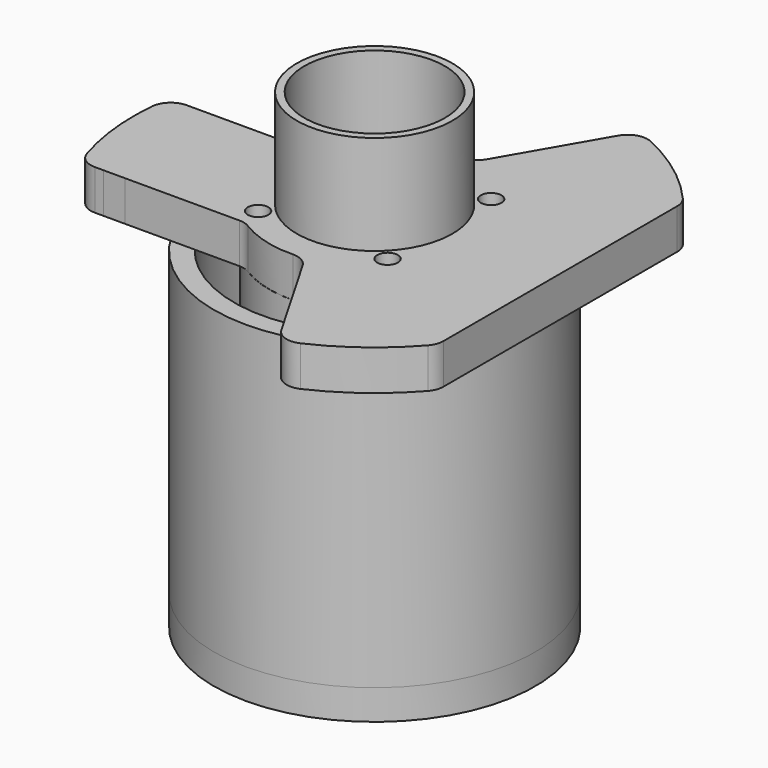
from build123d import *

# Parameters (mm, degrees)
F0_W      = 12.7
F0_H      = 12.86002
F0_R      = 11.1125
F0_H_2    = 0.00127
F1_DEPTH  = 6.35
F12_D     = 2.4384
F12_DEPTH = 4.7625
F12_TIP   = 0.7325692667
F11_R     = 21.63445
F11_R_2   = 14.478
F13_DEPTH = 1.190625
F14_D     = 2.4384
F16_D     = 2.2606
F16_DEPTH = 6.35
F16_TIP   = 0.6791527577
F17_D     = 3.2639


# Not quite as in the source:
# - a feature names something its author has since deleted; it is built from what else it names


with BuildPart() as f1:
    # F0 (on Top) → F1 (new body)
    with BuildSketch(Plane.XY):
        with BuildLine():
            ThreePointArc((29.36875, 23.1007161347), (29.1636905508, 24.2232481499), (28.575, 25.2007812379))
            ThreePointArc((28.575, 25.2007812379), (22.762711603, 30.5527242726), (15.9715205932, 34.5907578688))
            ThreePointArc((15.9715205932, 34.5907578688), (13.6801160021, 34.7344417755), (11.8909298868, 33.2956947131))
            Line((11.8909298868, 33.2956947131), (3.1737490765, 18.197094651))
            ThreePointArc((3.1737490765, 18.197094651), (1.9820606936, 17.0181093591), (0.3560722092, 16.6103239138))
            ThreePointArc((0.3560722092, 16.6103239138), (-8.30707, 14.388267302), (-14.5629985791, 7.9967943781))
            ThreePointArc((-14.5629985791, 7.9967943781), (-15.7291453761, 6.792539767), (-17.3460207811, 6.35))
            Line((-17.3460207811, 6.35), (-34.7803824016, 6.35))
            ThreePointArc((-34.7803824016, 6.35), (-36.9209669649, 5.5198929032), (-37.9422353472, 3.4636363636))
            ThreePointArc((-37.9422353472, 3.4636363636), (-37.8826451562, -4.0638892662), (-36.3442120473, -11.4327709091))
            ThreePointArc((-36.3442120473, -11.4327709091), (-35.1937854617, -13.039878436), (-33.31552771, -13.65504))
            Line((-33.31552771, -13.65504), (-31.9626256824, -13.65377))
            Line((-31.9626256824, -13.65377), (-28.575, -13.65377))
            Line((-28.575, -13.65377), (-28.575, -6.35))
            Line((-28.575, -6.35), (-28.575, -0.79375))
            Line((-28.575, -0.79375), (-15.875, -0.79375))
            Line((-15.875, -0.79375), (-15.875, -13.65377))
            Line((-15.875, -13.65377), (-15.875, -13.65504))
            Line((-15.875, -13.65504), (-10.4096020836, -13.65504))
            ThreePointArc((-10.4096020836, -13.65504), (-9.5414514384, -13.7760361596), (-8.7394695454, -14.1298025465))
            ThreePointArc((-8.7394695454, -14.1298025465), (-4.3713366706, -16.0287573958), (0.3560722092, -16.6103239138))
            ThreePointArc((0.3560722092, -16.6103239138), (1.9820606936, -17.0181093591), (3.1737490765, -18.197094651))
            Line((3.1737490765, -18.197094651), (11.8909298868, -33.2956947131))
            ThreePointArc((11.8909298868, -33.2956947131), (13.6801160021, -34.7344417755), (15.9715205932, -34.5907578688))
            ThreePointArc((15.9715205932, -34.5907578688), (22.762711603, -30.5527242726), (28.575, -25.2007812379))
            ThreePointArc((28.575, -25.2007812379), (29.1636905508, -24.2232481499), (29.36875, -23.1007161347))
            Line((29.36875, -23.1007161347), (29.36875, 23.1007161347))
        make_face()
        with Locations((22.225, -7.22376)):
            Rectangle(F0_W, F0_H, mode=Mode.SUBTRACT)
        Circle(F0_R, mode=Mode.SUBTRACT)
        with Locations((-22.225, -13.654405)):
            Rectangle(F0_W, F0_H_2)
        Polygon((-28.575, -13.65377), (-15.875, -13.65377), (-15.875, -0.79375), (-28.575, -0.79375), (-28.575, -6.35), align=None)
        with Locations((22.225, -7.22376)):
            Rectangle(F0_W, F0_H)
    extrude(amount=F1_DEPTH)

    # F17 (through all)
    with Locations(Plane(origin=(0, 0, 0), x_dir=(1, 0, 0), z_dir=(0, 0, -1))):
        with Locations((-10.237491978, -10.237491978), (10.237491978, -10.237491978), (10.237491978, 10.237491978), (-10.237491978, 10.237491978)):
            Hole(F17_D / 2)


with BuildPart() as f6:
    # F5 (on Right) → F6 (revolve)
    with BuildSketch(Plane.YZ):
        Polygon((12.303125, 22.08276), (11.1125, 22.08276), (11.1125, -26.91638), (13.462, -26.91638), (13.462, -25.725755), (12.303125, -25.725755), align=None)
    revolve(axis=Axis((0, 0, -24.5783533533), (0, 0, -1)))


with BuildPart() as f8:
    # F7 (on Right) → F8 (revolve)
    with BuildSketch(Plane.YZ):
        with BuildLine():
            Line((13.462, -25.725755), (13.462, -26.91638))
            Line((13.462, -26.91638), (13.462, -49.2125))
            Line((13.462, -49.2125), (14.1478, -49.2125))
            ThreePointArc((14.1478, -49.2125), (15.0368, -48.3235), (15.9258, -49.2125))
            Line((15.9258, -49.2125), (16.891, -49.2125))
            Line((16.891, -49.2125), (16.891, -52.3875))
            Line((16.891, -52.3875), (25.4, -52.3875))
            Line((25.4, -52.3875), (25.4, -47.625))
            Line((25.4, -47.625), (22.225, -47.625))
            Line((22.225, -47.625), (22.225, -42.8625))
            Line((22.225, -42.8625), (16.637, -42.8625))
            Line((16.637, -42.8625), (16.637, 0))
            Line((16.637, 0), (12.303125, 0))
            Line((12.303125, 0), (12.303125, -25.725755))
            Line((12.303125, -25.725755), (13.462, -25.725755))
        make_face()
    revolve(axis=Axis((0, 0, -24.60625), (0, 0, -1)))

    # F12
    with Locations(Plane(origin=(0, 0, -52.3875), x_dir=(1, 0, 0), z_dir=(0, 0, -1))):
        with Locations((-18.4785, 0), (9.23925, 16.0028504238), (18.4785, 0), (9.23925, -16.0028504238), (-9.23925, -16.0028504238), (-9.23925, 16.0028504238)):
            Hole(F12_D / 2, depth=F12_DEPTH)
            with Locations((0, 0, -(F12_DEPTH + F12_TIP / 2))):  # 118° drill point
                Cone(0, F12_D / 2, F12_TIP, mode=Mode.SUBTRACT)

    # F16
    with Locations(Plane.XY):
        with Locations((-10.237491978, 10.237491978), (10.237491978, 10.237491978), (10.237491978, -10.237491978), (-10.237491978, -10.237491978)):
            Hole(F16_D / 2, depth=F16_DEPTH)
            with Locations((0, 0, -(F16_DEPTH + F16_TIP / 2))):  # 118° drill point
                Cone(0, F16_D / 2, F16_TIP, mode=Mode.SUBTRACT)


with BuildPart() as f10:
    # F9 (on Right) → F10 (revolve)
    with BuildSketch(Plane.YZ):
        Polygon((22.225, -42.8625), (22.225, -47.625), (25.4, -47.625), (25.4, 0), (22.225, 0), align=None)
    revolve(axis=Axis((0, 0, -24.60625), (0, 0, -1)))


with BuildPart() as f13:
    # F11 (on face) → F13 (new body)
    with BuildSketch(Plane(origin=(0, 0, -52.3875), x_dir=(1, 0, 0), z_dir=(0, 0, -1))):
        Circle(F11_R)
        Circle(F11_R_2, mode=Mode.SUBTRACT)
    extrude(amount=F13_DEPTH)

    # F14 (through all)
    with Locations(Plane.XY.offset(-52.3875)):
        with Locations((9.23925, -16.0028504238), (18.4785, 0), (9.23925, 16.0028504238), (-9.23925, 16.0028504238), (-18.4785, 0), (-9.23925, -16.0028504238)):
            Hole(F14_D / 2)


solid = Compound([f1.part, f6.part, f8.part, f10.part, f13.part])
